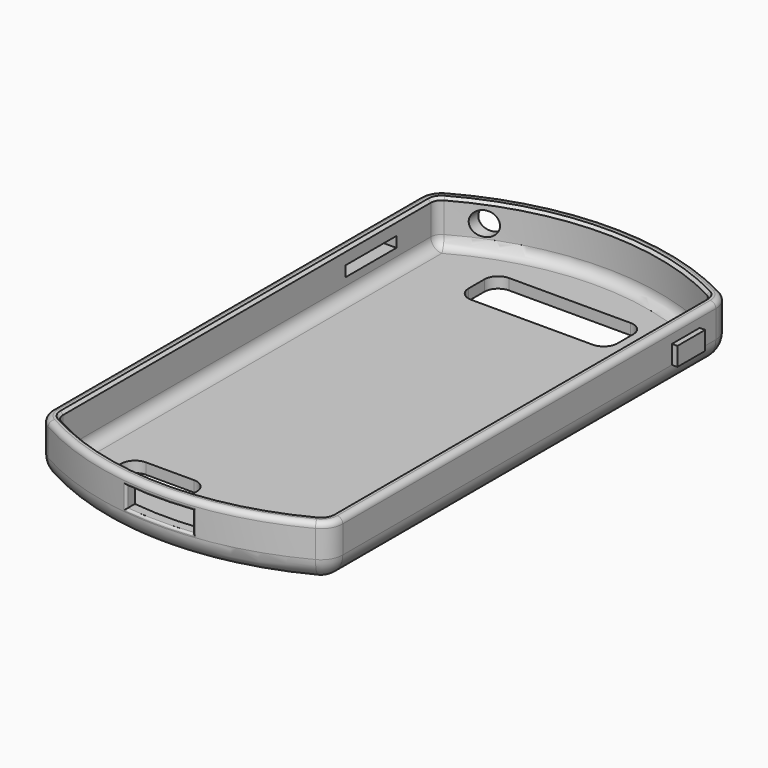
from build123d import *

# Parameters (mm, degrees)
F1_DEPTH     = 12.7
F2_R         = 5.08
F3_T         = -2.54
F4_SIZE      = 0.635
F5_R         = 1.27
F6_W         = 15.4954232275
F6_H         = 4.7704899881
F7_DEPTH     = 66.1637644998
F8_T1_DEPTH  = 4.7704899881
F8_T6_ANGLE  = 15.6492345412
F8_T12_ANGLE = 15.6492345412
F8_T19_ANGLE = 15.6492345412
F8_T23_DEPTH = 6.2108427353
F8_T30_ANGLE = 15.6492345412
F8_T34_DEPTH = 6.2108427353
F8_T41_ANGLE = 15.6492345412
F8_T45_DEPTH = 6.2108427353
F8_T52_DEPTH = 6.2108427353
F8_T56_ANGLE = 15.6492345412
F9_W         = 8.0456919968
F9_H         = 4.306647027
F10_DEPTH    = 1.27
F11_R        = 2.7398291671
F12_DEPTH    = 66.1637645998
F13_W        = 16.0913988948
F13_H        = 3.5758665763
F14_DEPTH    = 1.27
F16_DEPTH    = 12.701
F18_DEPTH    = 12.701
F19_W        = 14.7827621549
F19_H        = 2.4444661103
F20_DEPTH    = 35.56
F21_W        = 6.5305903554
F21_H        = 2.8003924526
F22_DEPTH    = 34.29


# Not quite as in the source:
# - a fillet or chamfer that OpenCascade refuses, or shapes differently, is made with other operations: its cross-section is extruded or revolved along the edge and cut away or added


with BuildPart() as f1:
    # F0 (on Top) → F1 (new body)
    with BuildSketch(Plane.XY):
        with BuildLine():
            Line((33.3375, -57.15), (33.3375, 57.15))
            ThreePointArc((33.3375, 57.15), (-0.8382267858, 66.1574544712), (-34.7747671557, 56.2870053877))
            Line((-34.7747671557, 56.2870053877), (-34.7747671557, -56.2870053877))
            ThreePointArc((-34.7747671557, -56.2870053877), (-0.8382267858, -66.1574544712), (33.3375, -57.15))
        make_face()
    extrude(amount=F1_DEPTH)

    # F2
    f2_edges = [f1.edges().sort_by_distance(p)[0] for p in [
        (33.3375, -57.15, 6.35),
        (33.3375, 0, 0),
        (-34.774767, 0, 0),
        (-0.838227, 66.157454, 0),
        (-34.774767, 56.287005, 6.35),
        (33.3375, 57.15, 6.35),
        (-0.838227, -66.157454, 0),
        (-34.774767, -56.287005, 6.35),
    ]]
    fillet(f2_edges, radius=F2_R)

    # F3
    f3_openings = [f1.faces().sort_by_distance(p)[0] for p in [
        (-0.646739, 0, 12.7),
    ]]
    offset(amount=F3_T, openings=f3_openings)

    # F4
    f4_edges = [f1.edges().sort_by_distance(p)[0] for p in [
        (-0.850297, 63.617082, 12.7),
        (30.7975, 0, 12.7),
        (-0.850297, -63.617082, 12.7),
        (-32.234767, 0, 12.7),
        (-31.884285, 54.66655, 12.7),
        (30.429616, 55.470279, 12.7),
        (30.429616, -55.470279, 12.7),
        (-31.884285, -54.66655, 12.7),
    ]]
    chamfer(f4_edges, length=F4_SIZE)

    # F5
    f5_edges = [f1.edges().sort_by_distance(p)[0] for p in [
        (33.3375, 0, 12.7),
        (32.601732, -56.786909, 12.7),
        (-0.884243, -66.156855, 12.7),
        (-34.073804, -55.954032, 12.7),
        (-34.774767, 0, 12.7),
        (-34.073804, 55.954032, 12.7),
        (-0.884243, 66.156855, 12.7),
        (32.601732, 56.786909, 12.7),
    ]]
    fillet(f5_edges, radius=F5_R)

    # F6 (on Front) → F7 (cut, through all)
    with BuildSketch(Plane.XZ):
        with Locations((0, 8.1946933642)):
            Rectangle(F6_W, F6_H)
    extrude(amount=F7_DEPTH, mode=Mode.SUBTRACT)

    # F8: fillet of radius 0.508 on 4 edges, made by hand

    # F8_s2 → F8_t1 (cut)
    with BuildSketch(Plane.XY.offset(5.8094483702)):
        with BuildLine():
            ThreePointArc((-8.3195897121, -65.6376098991), (-7.9198441354, -65.5147680663), (-7.7477116138, -65.1336420544))
            Line((-7.7477116138, -65.1336420544), (-7.7477116138, -65.7075670756))
            ThreePointArc((-7.7477116138, -65.7075670756), (-8.0337268111, -65.6732109751), (-8.3195897121, -65.6376098991))
        make_face()
        with BuildLine():
            ThreePointArc((8.3195897121, -65.6376098991), (7.9198441354, -65.5147680663), (7.7477116138, -65.1336420544))
            Line((7.7477116138, -65.1336420544), (7.7477116138, -65.7075670756))
            ThreePointArc((7.7477116138, -65.7075670756), (8.0337268111, -65.6732109751), (8.3195897121, -65.6376098991))
        make_face()
    extrude(amount=F8_T1_DEPTH, mode=Mode.SUBTRACT)


with BuildPart() as f8_tool4:
    # F8_s5 → F8_t6 (revolve)
    with BuildSketch(Plane(origin=(0, 0, 0), x_dir=(0, 0, 1), z_dir=(0.9906894385, 0.1361412371, 0))):
        with BuildLine():
            ThreePointArc((5.3014483702, 66.1627644998), (5.660658615, 66.0139747446), (5.8094483702, 65.6547644998))
            Line((5.8094483702, 65.6547644998), (5.8094483702, 66.1627644998))
            Line((5.8094483702, 66.1627644998), (5.3014483702, 66.1627644998))
        make_face()
    revolve(axis=Axis((0, 0, 5.8094483702), (0, 0, -1)), revolution_arc=F8_T6_ANGLE)

    split(bisect_by=Plane.YZ.offset(7.7477116138), keep=Keep.BOTTOM)

    split(bisect_by=Plane.YZ.offset(-7.7477116138), keep=Keep.TOP)


with BuildPart() as f1_1:
    add(f1.part)

    # F8_t3: cut F8_tool4
    add(f8_tool4.part, mode=Mode.SUBTRACT)


with BuildPart() as f8_tool10:
    # F8_s11 → F8_t12 (revolve)
    with BuildSketch(Plane(origin=(0, 0, 0), x_dir=(0, 0, 1), z_dir=(0.9906894385, 0.1361412371, 0))):
        with BuildLine():
            ThreePointArc((11.0879383582, 66.1627644998), (10.7287281134, 66.0139747446), (10.5799383582, 65.6547644998))
            Line((10.5799383582, 65.6547644998), (10.5799383582, 66.1627644998))
            Line((10.5799383582, 66.1627644998), (11.0879383582, 66.1627644998))
        make_face()
    revolve(axis=Axis((0, 0, 10.5799383582), (0, 0, -1)), revolution_arc=F8_T12_ANGLE)

    split(bisect_by=Plane.YZ.offset(-7.7477116138), keep=Keep.TOP)

    split(bisect_by=Plane.YZ.offset(7.7477116138), keep=Keep.BOTTOM)


with BuildPart() as f1_2:
    add(f1_1.part)

    # F8_t9: cut F8_tool10
    add(f8_tool10.part, mode=Mode.SUBTRACT)


with BuildPart() as f8_tool17:
    # F8_s18 → F8_t19 (revolve)
    with BuildSketch(Plane(origin=(0, 0, 0), x_dir=(0, 0, 1), z_dir=(0.9906894385, 0.1361412371, 0))):
        with BuildLine():
            ThreePointArc((11.0879383582, 66.1627644998), (10.7287281134, 66.0139747446), (10.5799383582, 65.6547644998))
            Line((10.5799383582, 65.6547644998), (10.5799383582, 66.1627644998))
            Line((10.5799383582, 66.1627644998), (11.0879383582, 66.1627644998))
        make_face()
    revolve(axis=Axis((0, 0, 10.5799383582), (0, 0, -1)), revolution_arc=F8_T19_ANGLE)

    split(bisect_by=Plane.YZ.offset(-7.7477116138), keep=Keep.BOTTOM)


with BuildPart() as f8_tool21:
    # F8_s22 → F8_t23 (new body)
    with BuildSketch(Plane.XY.offset(12.0202911055)):
        with BuildLine():
            ThreePointArc((-8.3195897121, -65.6376098991), (-7.9198441354, -65.5147680663), (-7.7477116138, -65.1336420544))
            Line((-7.7477116138, -65.1336420544), (-7.7477116138, -65.7075670756))
            ThreePointArc((-7.7477116138, -65.7075670756), (-8.0337268111, -65.6732109751), (-8.3195897121, -65.6376098991))
        make_face()
    extrude(amount=-F8_T23_DEPTH)

    split(bisect_by=Plane.XY.offset(10.5799383582), keep=Keep.TOP)


with BuildPart() as f8_tool17_1:
    add(f8_tool17.part)

    # F8_t25: intersect F8_tool21
    add(f8_tool21.part, mode=Mode.INTERSECT)


with BuildPart() as f1_3:
    add(f1_2.part)

    # F8_t15: cut F8_tool17
    add(f8_tool17_1.part, mode=Mode.SUBTRACT)


with BuildPart() as f8_tool28:
    # F8_s29 → F8_t30 (revolve)
    with BuildSketch(Plane(origin=(0, 0, 0), x_dir=(0, 0, 1), z_dir=(0.9906894385, 0.1361412371, 0))):
        with BuildLine():
            ThreePointArc((5.3014483702, 66.1627644998), (5.660658615, 66.0139747446), (5.8094483702, 65.6547644998))
            Line((5.8094483702, 65.6547644998), (5.8094483702, 66.1627644998))
            Line((5.8094483702, 66.1627644998), (5.3014483702, 66.1627644998))
        make_face()
    revolve(axis=Axis((0, 0, 5.8094483702), (0, 0, -1)), revolution_arc=F8_T30_ANGLE)

    split(bisect_by=Plane.YZ.offset(-7.7477116138), keep=Keep.BOTTOM)


with BuildPart() as f8_tool32:
    # F8_s33 → F8_t34 (new body)
    with BuildSketch(Plane.XY.offset(10.5799383582)):
        with BuildLine():
            ThreePointArc((-8.3195897121, -65.6376098991), (-7.9198441354, -65.5147680663), (-7.7477116138, -65.1336420544))
            Line((-7.7477116138, -65.1336420544), (-7.7477116138, -65.7075670756))
            ThreePointArc((-7.7477116138, -65.7075670756), (-8.0337268111, -65.6732109751), (-8.3195897121, -65.6376098991))
        make_face()
    extrude(amount=-F8_T34_DEPTH)

    split(bisect_by=Plane.XY.offset(5.8094483702), keep=Keep.BOTTOM)


with BuildPart() as f8_tool28_1:
    add(f8_tool28.part)

    # F8_t36: intersect F8_tool32
    add(f8_tool32.part, mode=Mode.INTERSECT)


with BuildPart() as f1_4:
    add(f1_3.part)

    # F8_t26: cut F8_tool28
    add(f8_tool28_1.part, mode=Mode.SUBTRACT)


with BuildPart() as f8_tool39:
    # F8_s40 → F8_t41 (revolve)
    with BuildSketch(Plane(origin=(0, 0, 0), x_dir=(0, 0, 1), z_dir=(0.9906894385, 0.1361412371, 0))):
        with BuildLine():
            ThreePointArc((11.0879383582, 66.1627644998), (10.7287281134, 66.0139747446), (10.5799383582, 65.6547644998))
            Line((10.5799383582, 65.6547644998), (10.5799383582, 66.1627644998))
            Line((10.5799383582, 66.1627644998), (11.0879383582, 66.1627644998))
        make_face()
    revolve(axis=Axis((0, 0, 10.5799383582), (0, 0, -1)), revolution_arc=F8_T41_ANGLE)

    split(bisect_by=Plane.YZ.offset(7.7477116138), keep=Keep.TOP)


with BuildPart() as f8_tool43:
    # F8_s44 → F8_t45 (new body)
    with BuildSketch(Plane.XY.offset(12.0202911055)):
        with BuildLine():
            ThreePointArc((8.3195897121, -65.6376098991), (7.9198441354, -65.5147680663), (7.7477116138, -65.1336420544))
            Line((7.7477116138, -65.1336420544), (7.7477116138, -65.7075670756))
            ThreePointArc((7.7477116138, -65.7075670756), (8.0337268111, -65.6732109751), (8.3195897121, -65.6376098991))
        make_face()
    extrude(amount=-F8_T45_DEPTH)

    split(bisect_by=Plane.XY.offset(10.5799383582), keep=Keep.TOP)


with BuildPart() as f8_tool39_1:
    add(f8_tool39.part)

    # F8_t47: intersect F8_tool43
    add(f8_tool43.part, mode=Mode.INTERSECT)


with BuildPart() as f1_5:
    add(f1_4.part)

    # F8_t37: cut F8_tool39
    add(f8_tool39_1.part, mode=Mode.SUBTRACT)


with BuildPart() as f8_tool50:
    # F8_s51 → F8_t52 (new body)
    with BuildSketch(Plane.XY.offset(10.5799383582)):
        with BuildLine():
            ThreePointArc((8.3195897121, -65.6376098991), (7.9198441354, -65.5147680663), (7.7477116138, -65.1336420544))
            Line((7.7477116138, -65.1336420544), (7.7477116138, -65.7075670756))
            ThreePointArc((7.7477116138, -65.7075670756), (8.0337268111, -65.6732109751), (8.3195897121, -65.6376098991))
        make_face()
    extrude(amount=-F8_T52_DEPTH)

    split(bisect_by=Plane.XY.offset(5.8094483702), keep=Keep.BOTTOM)


with BuildPart() as f8_tool54:
    # F8_s55 → F8_t56 (revolve)
    with BuildSketch(Plane(origin=(0, 0, 0), x_dir=(0, 0, 1), z_dir=(0.9906894385, 0.1361412371, 0))):
        with BuildLine():
            ThreePointArc((5.3014483702, 66.1627644998), (5.660658615, 66.0139747446), (5.8094483702, 65.6547644998))
            Line((5.8094483702, 65.6547644998), (5.8094483702, 66.1627644998))
            Line((5.8094483702, 66.1627644998), (5.3014483702, 66.1627644998))
        make_face()
    revolve(axis=Axis((0, 0, 5.8094483702), (0, 0, -1)), revolution_arc=F8_T56_ANGLE)

    split(bisect_by=Plane.YZ.offset(7.7477116138), keep=Keep.TOP)


with BuildPart() as f8_tool50_1:
    add(f8_tool50.part)

    # F8_t58: intersect F8_tool54
    add(f8_tool54.part, mode=Mode.INTERSECT)


with BuildPart() as f1_6:
    add(f1_5.part)

    # F8_t48: cut F8_tool50
    add(f8_tool50_1.part, mode=Mode.SUBTRACT)

    # F9 (on face) → F10 (join)
    with BuildSketch(Plane.YZ.offset(33.3375)):
        with Locations((45.4432945698, 7.2333235135)):
            Rectangle(F9_W, F9_H)
    extrude(amount=F10_DEPTH)

    # F11 (on Front) → F12 (cut, through all)
    with BuildSketch(Plane.XZ):
        with Locations((-24.1370927542, 8.1946933642)):
            Circle(F11_R)
    extrude(amount=-F12_DEPTH, mode=Mode.SUBTRACT)

    # F13 (on face) → F14 (join)
    with BuildSketch(Plane(origin=(-34.7747671557, 0, 0), x_dir=(0, -1, 0), z_dir=(-1, 0, 0))):
        with Locations((-36.0566489398, 8.1946933642)):
            Rectangle(F13_W, F13_H)
    extrude(amount=F14_DEPTH)

    # F15 (on face) → F16 (cut, through all)
    with BuildSketch(Plane(origin=(0, 0, 0), x_dir=(1, 0, 0), z_dir=(0, 0, -1))):
        with BuildLine():
            Line((-14.1083539546, -53.4263903977), (14.1083539546, -53.4263903977))
            ThreePointArc((14.1083539546, -53.4263903977), (16.3534179848, -52.4964544279), (17.2833539546, -50.2513903977))
            Line((17.2833539546, -50.2513903977), (17.2833539546, -45.6384069204))
            ThreePointArc((17.2833539546, -45.6384069204), (16.3534179848, -43.3933428902), (14.1083539546, -42.4634069204))
            Line((14.1083539546, -42.4634069204), (-14.1083539546, -42.4634069204))
            ThreePointArc((-14.1083539546, -42.4634069204), (-16.3534179848, -43.3933428902), (-17.2833539546, -45.6384069204))
            Line((-17.2833539546, -45.6384069204), (-17.2833539546, -50.2513903977))
            ThreePointArc((-17.2833539546, -50.2513903977), (-16.3534179848, -52.4964544279), (-14.1083539546, -53.4263903977))
        make_face()
    extrude(amount=-F16_DEPTH, mode=Mode.SUBTRACT)

    # F17 (on face) → F18 (cut, through all)
    with BuildSketch(Plane(origin=(0, 0, 0), x_dir=(1, 0, 0), z_dir=(0, 0, -1))):
        with BuildLine():
            Line((-20.30652088, 44.2513413727), (-9.1347757645, 44.2513413727))
            ThreePointArc((-9.1347757645, 44.2513413727), (-6.8897117342, 45.1812773425), (-5.9597757645, 47.4263413727))
            Line((-5.9597757645, 47.4263413727), (-5.9597757645, 49.4200230658))
            ThreePointArc((-5.9597757645, 49.4200230658), (-6.8897117342, 51.6650870961), (-9.1347757645, 52.5950230658))
            Line((-9.1347757645, 52.5950230658), (-20.30652088, 52.5950230658))
            ThreePointArc((-20.30652088, 52.5950230658), (-22.5515849103, 51.6650870961), (-23.48152088, 49.4200230658))
            Line((-23.48152088, 49.4200230658), (-23.48152088, 47.4263413727))
            ThreePointArc((-23.48152088, 47.4263413727), (-22.5515849103, 45.1812773425), (-20.30652088, 44.2513413727))
        make_face()
    extrude(amount=-F18_DEPTH, mode=Mode.SUBTRACT)

    # F19 (on Right) → F20 (cut)
    with BuildSketch(Plane.YZ):
        with Locations((36.0044911504, 8.1135937944)):
            Rectangle(F19_W, F19_H)
    extrude(amount=-F20_DEPTH, mode=Mode.SUBTRACT)

    # F21 (on Right) → F22 (cut)
    with BuildSketch(Plane.YZ):
        with Locations((45.5593243241, 7.3050209321)):
            Rectangle(F21_W, F21_H)
    extrude(amount=F22_DEPTH, mode=Mode.SUBTRACT)


solid = f1_6.part
